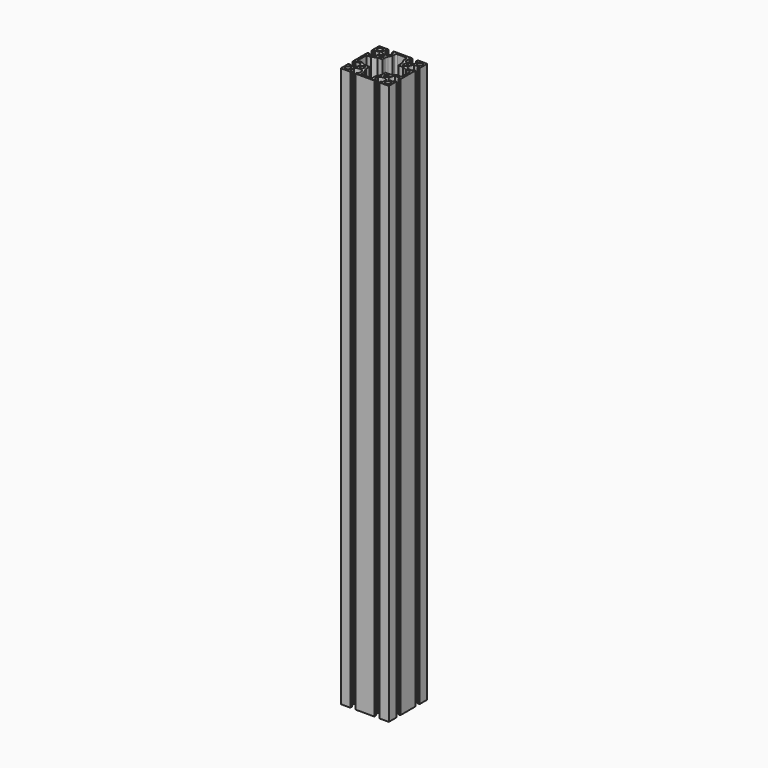
from build123d import *

# Parameters (mm, degrees)
F0_R     = 3
F0_R_2   = 2.5
F1_DEPTH = 700
F2_R     = 2
F3_R     = 7


# Not quite as in the source:
# - a feature names something its author has since deleted; it is built from what else it names


with BuildPart() as f1:
    # F0 (on Top) → F1 (new body)
    with BuildSketch(Plane.XY):
        with BuildLine():
            Line((18.15, -30), (30, -30))
            Line((30, -30), (30, -18.15))
            Line((30, -18.15), (27.5, -18.15))
            Line((27.5, -18.15), (27.5, -20.15))
            Line((27.5, -20.15), (21.5477069044, -20.15))
            ThreePointArc((21.5477069044, -20.15), (19.5, -15), (21.5477069044, -9.85))
            Line((21.5477069044, -9.85), (27.5, -9.85))
            Line((27.5, -9.85), (27.5, -11.85))
            Line((27.5, -11.85), (30, -11.85))
            Line((30, -11.85), (30, 11.85))
            Line((30, 11.85), (27.5, 11.85))
            Line((27.5, 11.85), (27.5, 9.85))
            Line((27.5, 9.85), (21.5477069044, 9.85))
            ThreePointArc((21.5477069044, 9.85), (19.5, 15), (21.5477069044, 20.15))
            Line((21.5477069044, 20.15), (27.5, 20.15))
            Line((27.5, 20.15), (27.5, 18.15))
            Line((27.5, 18.15), (30, 18.15))
            Line((30, 18.15), (30, 30))
            Line((30, 30), (18.15, 30))
            Line((18.15, 30), (18.15, 27.5))
            Line((18.15, 27.5), (20.15, 27.5))
            Line((20.15, 27.5), (20.15, 21.5477069044))
            ThreePointArc((20.15, 21.5477069044), (15, 19.5), (9.85, 21.5477069044))
            Line((9.85, 21.5477069044), (9.85, 27.5))
            Line((9.85, 27.5), (11.85, 27.5))
            Line((11.85, 27.5), (11.85, 30))
            Line((11.85, 30), (-11.85, 30))
            Line((-11.85, 30), (-11.85, 27.5))
            Line((-11.85, 27.5), (-9.85, 27.5))
            Line((-9.85, 27.5), (-9.85, 21.5477069044))
            ThreePointArc((-9.85, 21.5477069044), (-15, 19.5), (-20.15, 21.5477069044))
            Line((-20.15, 21.5477069044), (-20.15, 27.5))
            Line((-20.15, 27.5), (-18.15, 27.5))
            Line((-18.15, 27.5), (-18.15, 30))
            Line((-18.15, 30), (-30, 30))
            Line((-30, 30), (-30, 18.15))
            Line((-30, 18.15), (-27.5, 18.15))
            Line((-27.5, 18.15), (-27.5, 20.15))
            Line((-27.5, 20.15), (-21.5477069044, 20.15))
            ThreePointArc((-21.5477069044, 20.15), (-19.5, 15), (-21.5477069044, 9.85))
            Line((-21.5477069044, 9.85), (-27.5, 9.85))
            Line((-27.5, 9.85), (-27.5, 11.85))
            Line((-27.5, 11.85), (-30, 11.85))
            Line((-30, 11.85), (-30, -11.85))
            Line((-30, -11.85), (-27.5, -11.85))
            Line((-27.5, -11.85), (-27.5, -9.85))
            Line((-27.5, -9.85), (-21.5477069044, -9.85))
            ThreePointArc((-21.5477069044, -9.85), (-19.5, -15), (-21.5477069044, -20.15))
            Line((-21.5477069044, -20.15), (-27.5, -20.15))
            Line((-27.5, -20.15), (-27.5, -18.15))
            Line((-27.5, -18.15), (-30, -18.15))
            Line((-30, -18.15), (-30, -30))
            Line((-30, -30), (-18.15, -30))
            Line((-18.15, -30), (-18.15, -27.5))
            Line((-18.15, -27.5), (-20.15, -27.5))
            Line((-20.15, -27.5), (-20.15, -21.5477069044))
            ThreePointArc((-20.15, -21.5477069044), (-15, -19.5), (-9.85, -21.5477069044))
            Line((-9.85, -21.5477069044), (-9.85, -27.5))
            Line((-9.85, -27.5), (-11.85, -27.5))
            Line((-11.85, -27.5), (-11.85, -30))
            Line((-11.85, -30), (11.85, -30))
            Line((11.85, -30), (11.85, -27.5))
            Line((11.85, -27.5), (9.85, -27.5))
            Line((9.85, -27.5), (9.85, -21.5477069044))
            ThreePointArc((9.85, -21.5477069044), (15, -19.5), (20.15, -21.5477069044))
            Line((20.15, -21.5477069044), (20.15, -27.5))
            Line((20.15, -27.5), (18.15, -27.5))
            Line((18.15, -27.5), (18.15, -30))
        make_face()
        with Locations((-25, -25)):
            Circle(F0_R, mode=Mode.SUBTRACT)
        with Locations((-15, -15)):
            Circle(F0_R_2, mode=Mode.SUBTRACT)
        with Locations((25, -25)):
            Circle(F0_R, mode=Mode.SUBTRACT)
        with Locations((15, -15)):
            Circle(F0_R_2, mode=Mode.SUBTRACT)
        with Locations((-25, 25)):
            Circle(F0_R, mode=Mode.SUBTRACT)
        with Locations((-15, 15)):
            Circle(F0_R_2, mode=Mode.SUBTRACT)
        Polygon((-7, 22), (-7, 27.5), (0, 27.5), (7, 27.5), (7, 22), (10, 16), (10, 10), (16, 10), (22, 7), (27.5, 7), (27.5, 0), (27.5, -7), (22, -7), (16, -10), (10, -10), (10, -16), (7, -22), (7, -27.5), (0, -27.5), (-7, -27.5), (-7, -22), (-10, -16), (-10, -10), (-16, -10), (-22, -7), (-27.5, -7), (-27.5, 0), (-27.5, 7), (-22, 7), (-16, 10), (-10, 10), (-10, 16), align=None, mode=Mode.SUBTRACT)
        with Locations((15, 15)):
            Circle(F0_R_2, mode=Mode.SUBTRACT)
        with Locations((25, 25)):
            Circle(F0_R, mode=Mode.SUBTRACT)
    extrude(amount=F1_DEPTH)

    # F2
    f2_edges = [f1.edges().sort_by_distance(p)[0] for p in [
        (-7, 27.5, 350),
        (7, 27.5, 350),
    ]]
    fillet(f2_edges, radius=F2_R)

    # F3
    f3_edges = [f1.edges().sort_by_distance(p)[0] for p in [
        (-10, 16, 350),
        (10, 16, 350),
    ]]
    fillet(f3_edges, radius=F3_R)


solid = f1.part
